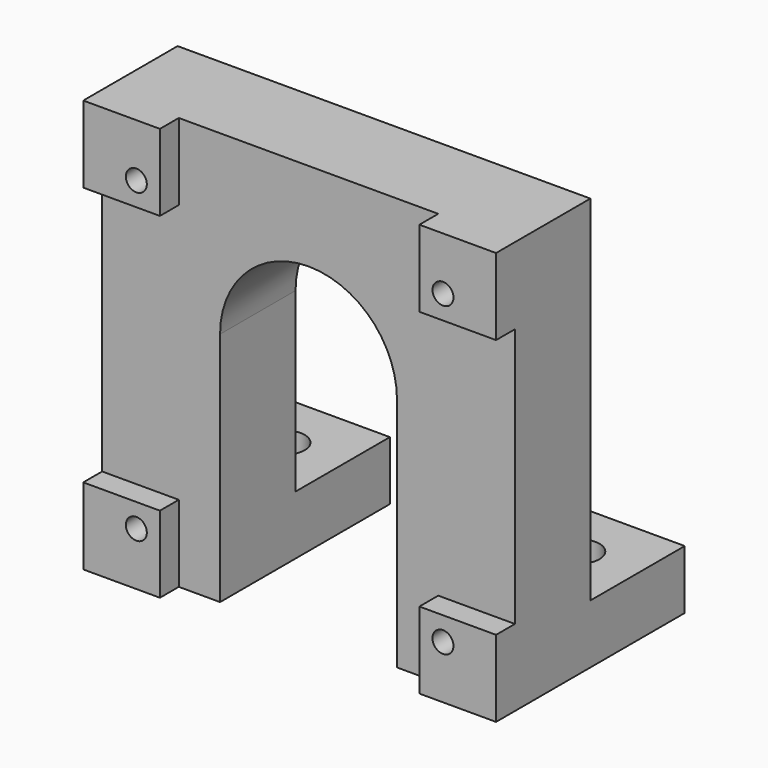
from build123d import *

# Parameters (mm, degrees)
F0_W     = 44.45
F0_H     = 44.45
F1_DEPTH = 12.7
F2_W     = 12.7
F2_H     = 6.35
F3_DEPTH = 12.7
F5_DEPTH = 2.54
F6_D     = 2.2606
F6_DEPTH = 11.43
F6_TIP   = 0.6791527577
F9_DEPTH = 12.701
F10_D    = 4.4958


# Not quite as in the source:
# - a pattern or mirror of a feature is missing from the dataset's text; its kind, count and spacing are read off the source's solid


with BuildPart() as f1:
    # F0 (on Front) → F1 (new body)
    with BuildSketch(Plane.XZ):
        Rectangle(F0_W, F0_H)
    extrude(amount=F1_DEPTH)

    # F2 (on face) → F3 (join)
    with BuildSketch(Plane(origin=(-22.225, 0, 0), x_dir=(0, -1, 0), z_dir=(-1, 0, 0))):
        with Locations((-6.35, -19.05)):
            Rectangle(F2_W, F2_H)
    f3 = extrude(amount=-F3_DEPTH)

    # F3_copies: F3 across plane
    add(f3.mirror(Plane(origin=(0, 0, 0), x_dir=(0, 0, 1), z_dir=(1, 0, 0))))

    # F4 (on face) → F5 (cut)
    with BuildSketch(Plane.XZ.offset(12.7)):
        Polygon((-13.97, 13.97), (-22.225, 13.97), (-22.225, 0), (-22.225, -13.97), (-13.97, -13.97), (-13.97, -22.225), (0, -22.225), (13.97, -22.225), (13.97, -13.97), (22.225, -13.97), (22.225, 0), (22.225, 13.97), (13.97, 13.97), (13.97, 22.225), (0, 22.225), (-13.97, 22.225), align=None)
    extrude(amount=-F5_DEPTH, mode=Mode.SUBTRACT)

    # F6
    with Locations(Plane.XZ.offset(12.7)):
        with Locations((-16.51, 16.51), (16.51, 16.51), (16.51, -16.51), (-16.51, -16.51)):
            Hole(F6_D / 2, depth=F6_DEPTH)
            with Locations((0, 0, -(F6_DEPTH + F6_TIP / 2))):  # 118° drill point
                Cone(0, F6_D / 2, F6_TIP, mode=Mode.SUBTRACT)

    # F8 (on face) → F9 (cut, through all)
    with BuildSketch(Plane(origin=(0, 0, 0), x_dir=(-1, 0, 0), z_dir=(0, 1, 0))):
        with BuildLine():
            Line((-9.525, 3.175), (-9.525, -22.225))
            Line((-9.525, -22.225), (9.525, -22.225))
            Line((9.525, -22.225), (9.525, 3.175))
            ThreePointArc((9.525, 3.175), (0, 12.7), (-9.525, 3.175))
        make_face()
    extrude(amount=-F9_DEPTH, mode=Mode.SUBTRACT)

    # F10 (through all)
    with Locations(Plane(origin=(0, 0, -22.225), x_dir=(1, 0, 0), z_dir=(0, 0, -1))):
        with Locations((15.875, -6.35)):
            f10 = Hole(F10_D / 2)

    # F10_copies: F10 across plane
    add(f10.mirror(Plane(origin=(0, 0, 0), x_dir=(0, 0, -1), z_dir=(-1, 0, 0))), mode=Mode.SUBTRACT)


solid = f1.part
